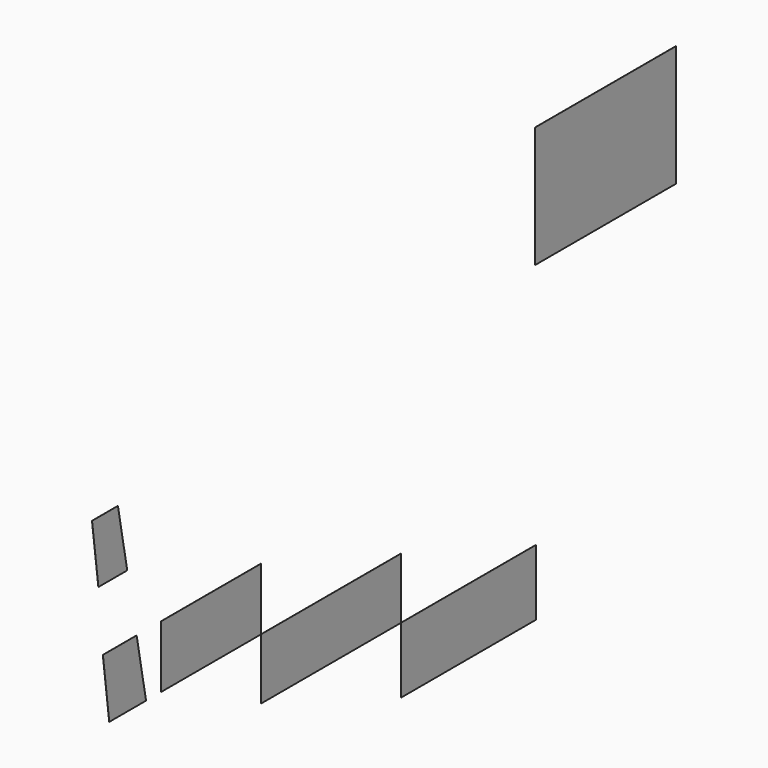
from build123d import *

# Parameters (mm, degrees)
F2_W     = 2786.5381240845
F2_H     = 1086.4863395691
F3_DEPTH = 1
F2_W_2   = 2877.9582977295
F2_H_2   = 1005.1188468933
F2_W_3   = 2058.3267211914
F2_H_3   = 1025.8510112762
F2_W_4   = 2907.6929092407
F2_H_4   = 1996.7029094696


with BuildPart() as f3:
    # F2 (on Right) → F3 (new body)
    with BuildSketch(Plane.YZ):
        with Locations((-12734.9848747253, -2574.2130279541)):
            Rectangle(F2_W, F2_H)
    extrude(amount=F3_DEPTH)


with BuildPart() as f3b:
    # F2 (on Right) → F3, piece 2 (new body)
    with BuildSketch(Plane.YZ):
        with Locations((-15567.2330856323, -1528.4104347229)):
            Rectangle(F2_W_2, F2_H_2)
    extrude(amount=F3_DEPTH)


with BuildPart() as f3c:
    # F2 (on Right) → F3, piece 3 (new body)
    with BuildSketch(Plane.YZ):
        with Locations((-18035.3755950928, -512.9255056381)):
            Rectangle(F2_W_3, F2_H_3)
    extrude(amount=F3_DEPTH)


with BuildPart() as f3d:
    # F2 (on Right) → F3, piece 4 (new body)
    with BuildSketch(Plane.YZ):
        Polygon((-19376.6774103795, -1025.8510112762), (-19570.8637237549, 0), (-20265.7604217529, 0), (-20134.6664428711, -1025.8510112762), align=None)
    extrude(amount=F3_DEPTH)


with BuildPart() as f3e:
    # F2 (on Right) → F3, piece 5 (new body)
    with BuildSketch(Plane.YZ):
        Polygon((-20358.1771850586, 1021.9507200357), (-19764.3117396887, 1021.9507200357), (-19956.2831208382, 2036.1006468002), (-20489.408493042, 2036.1006468002), align=None)
    extrude(amount=F3_DEPTH)


with BuildPart() as f3f:
    # F2 (on Right) → F3, piece 6 (new body)
    with BuildSketch(Plane.YZ):
        with Locations((-9912.9538536072, 3034.5431566238)):
            Rectangle(F2_W_4, F2_H_4)
    extrude(amount=F3_DEPTH)


solid = Compound([f3.part, f3b.part, f3c.part, f3d.part, f3e.part, f3f.part])
